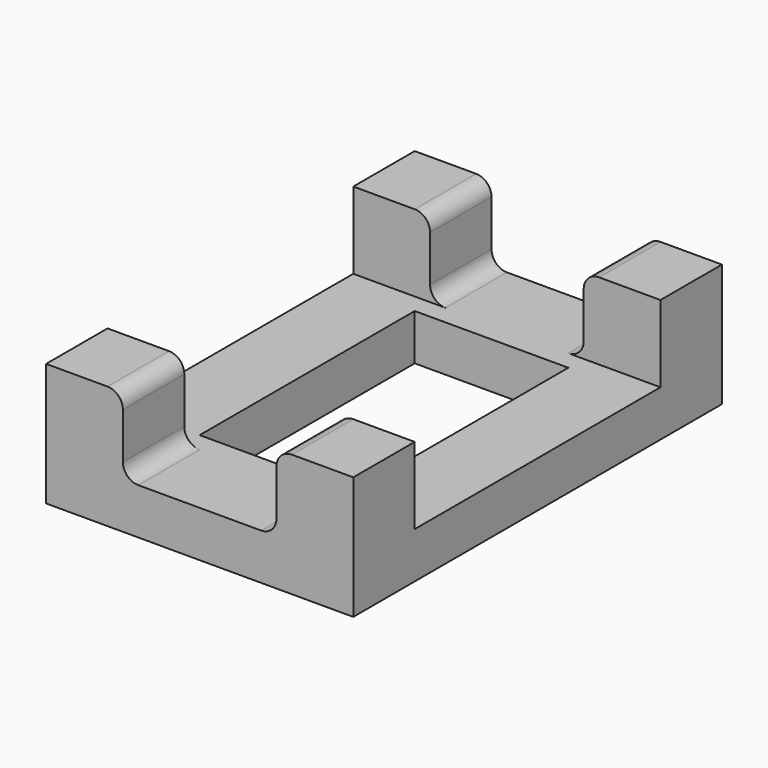
from build123d import *

# Parameters (mm, degrees)
F0_W      = 40
F0_H      = 60
F1_DEPTH  = 6
F2_W      = 10
F2_H      = 10
F3_DEPTH  = 10
F13_R     = 2
F14_W     = 20
F14_H     = 35
F15_DEPTH = 25


# Not quite as in the source:
# - the program builds the solid bodies; features that only make, move or delete a surface that nothing else refers to are left out


with BuildPart() as f1:
    # F0 (on Top) → F1 (new body)
    with BuildSketch(Plane.XY):
        Rectangle(F0_W, F0_H)
    extrude(amount=-F1_DEPTH)

    # F2 (on face) → F3 (join)
    with BuildSketch(Plane.XY):
        with Locations((-15, 25)):
            Rectangle(F2_W, F2_H)
        with Locations((15, 25)):
            Rectangle(F2_W, F2_H)
        with Locations((15, -25)):
            Rectangle(F2_W, F2_H)
        with Locations((-15, -25)):
            Rectangle(F2_W, F2_H)
    extrude(amount=F3_DEPTH)

    # F13
    f13_edges = [f1.edges().sort_by_distance(p)[0] for p in [
        (-10, 25, 10),
        (-10, -25, 10),
        (-10, -25, 0),
        (-10, 25, 0),
        (10, -25, 10),
        (10, 25, 10),
        (10, -25, 0),
        (10, 25, 0),
    ]]
    fillet(f13_edges, radius=F13_R)

    # F14 (on face) → F15 (cut)
    with BuildSketch(Plane.XY):
        Rectangle(F14_W, F14_H)
    extrude(amount=-F15_DEPTH, mode=Mode.SUBTRACT)


solid = f1.part
